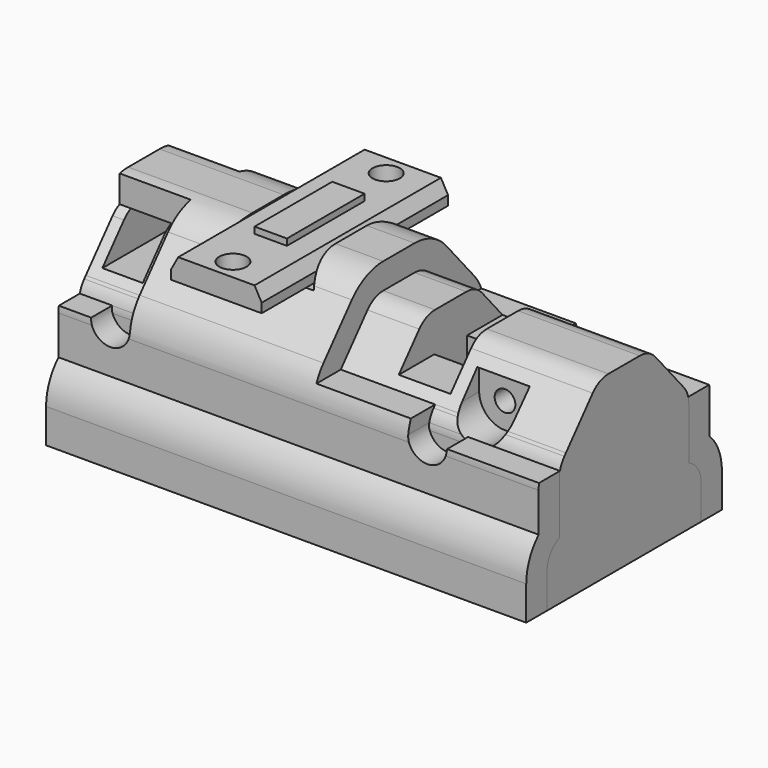
from build123d import *

# Parameters (mm, degrees)
F1_DEPTH    = 47.117
F2_T1_DEPTH = 58.7771515799
F2_T3_DEPTH = 56.5339110215
F2_T5_DEPTH = 65.2562282085
F3_T        = -2.54
F4_W        = 22.098
F4_H        = 12.7
F5_DEPTH    = 25.4
F7_DEPTH    = 25.4
F10_DEPTH   = 25.4
F12_DEPTH   = 25.4
F15_DEPTH   = 47.117
F16_W       = 3.9624000001
F16_H       = 3.9624
F17_DEPTH   = 25.4
F18_W       = 5.08
F18_H       = 6.35
F19_DEPTH   = 25.4
F20_R       = 1.016
F21_DEPTH   = 25.4
F23_R       = 1.016
F24_DEPTH   = 25.4
F26_DEPTH   = 25.4
F28_R       = 1.905
F29_DEPTH   = 25.4
F31_DEPTH   = 11.43
F32_W       = 1.5875
F32_H       = 0.635
F33_DEPTH   = 4.7625
F35_W       = 0.508
F35_H       = 2.1844
F36_DEPTH   = 12.7
F37_R       = 1.3462
F38_DEPTH   = 25.4


# Not quite as in the source:
# - a fillet or chamfer that OpenCascade refuses, or shapes differently, is made with other operations: its cross-section is extruded or revolved along the edge and cut away or added


with BuildPart() as f1:
    # F0 (on Right) → F1 (new body)
    with BuildSketch(Plane.YZ):
        Polygon((0, 6.985), (0, 0), (10.4775, 0), (12.0015, 0), (12.0015, 6.985), (10.4775, 6.985), (10.4775, 12.7), (4.2545, 19.939), (0, 19.939), align=None)
    extrude(amount=-F1_DEPTH)

    # F2: fillet of radius 5.08 on 3 edges, made by hand

    # F2_s2 → F2_t1 (cut)
    with BuildSketch(Plane.YZ.offset(-52.9470757899)):
        with BuildLine():
            ThreePointArc((5.7747186215, 18.1705824199), (4.0418518236, 19.4757758606), (1.922469684, 19.939))
            Line((1.922469684, 19.939), (4.2545, 19.939))
            Line((4.2545, 19.939), (5.7747186215, 18.1705824199))
        make_face()
    extrude(amount=F2_T1_DEPTH, mode=Mode.SUBTRACT)

    # F2_s4 → F2_t3 (cut)
    with BuildSketch(Plane.YZ.offset(-51.8254555107)):
        with BuildLine():
            ThreePointArc((9.2497489375, 14.1282002156), (10.160683001, 12.5825418311), (10.4775, 10.8166177957))
            Line((10.4775, 10.8166177957), (10.4775, 12.7))
            Line((10.4775, 12.7), (9.2497489375, 14.1282002156))
        make_face()
    extrude(amount=F2_T3_DEPTH, mode=Mode.SUBTRACT)

    # F2_s6 → F2_t5 (cut)
    with BuildSketch(Plane.YZ.offset(-56.1866141042)):
        with BuildLine():
            ThreePointArc((10.4775, 6.985), (11.6050285843, 5.3246298982), (12.0015, 3.3571543583))
            Line((12.0015, 3.3571543583), (12.0015, 6.985))
            Line((12.0015, 6.985), (10.4775, 6.985))
        make_face()
    extrude(amount=F2_T5_DEPTH, mode=Mode.SUBTRACT)

    # F3
    f3_openings = [f1.faces().sort_by_distance(p)[0] for p in [
        (0, 5.138779, 8.729827),
        (-23.5585, 0, 9.9695),
        (-47.117, 5.138779, 8.729827),
        (-23.5585, 6.00075, 0),
    ]]
    offset(amount=F3_T, openings=f3_openings, kind=Kind.INTERSECTION)

    # F4 (on Front) → F5 (cut)
    with BuildSketch(Plane.XZ):
        with Locations((-11.049, 19.05)):
            Rectangle(F4_W, F4_H)
    extrude(amount=-F5_DEPTH, mode=Mode.SUBTRACT)

    # F6 (on Front) → F7 (cut)
    with BuildSketch(Plane.XZ):
        with BuildLine():
            Line((-12.827, 17.78), (-12.827, 11.43))
            ThreePointArc((-12.827, 11.43), (-10.922, 9.525), (-9.017, 11.43))
            Line((-9.017, 11.43), (0, 11.43))
            Line((0, 11.43), (0, 17.78))
            Line((0, 17.78), (-10.922, 17.78))
            Line((-10.922, 17.78), (-12.827, 17.78))
        make_face()
    extrude(amount=-F7_DEPTH, mode=Mode.SUBTRACT)

    # F9 (on offset) → F10 (cut)
    with BuildSketch(Plane.XZ.offset(-2.9845)):
        with BuildLine():
            Line((-47.117, 11.43), (-43.942, 11.43))
            ThreePointArc((-43.942, 11.43), (-42.037, 9.525), (-40.132, 11.43))
            Line((-40.132, 11.43), (-40.132, 19.939))
            Line((-40.132, 19.939), (-42.037, 19.939))
            Line((-42.037, 19.939), (-47.117, 19.939))
            Line((-47.117, 19.939), (-47.117, 17.399))
            Line((-47.117, 17.399), (-47.117, 11.43))
        make_face()
    extrude(amount=-F10_DEPTH, mode=Mode.SUBTRACT)

    # F11 (on Front) → F12 (cut)
    with BuildSketch(Plane.XZ):
        Polygon((-26.7803559926, 19.939), (-34.9416440074, 19.939), (-36.068, 17.907), (-25.654, 17.907), align=None)
    extrude(amount=-F12_DEPTH, mode=Mode.SUBTRACT)

    # F13: F1 across plane


with BuildPart() as f1_1:
    add(f1.part)
    add(f1.part.mirror(Plane.XZ))


with BuildPart() as f15:
    # F14 (on Right) → F15 (new body, through all)
    with BuildSketch(Plane.YZ):
        with BuildLine():
            ThreePointArc((3.8485941527, 16.51479121), (2.9821607538, 17.1673879303), (1.922469684, 17.399))
            Line((1.922469684, 17.399), (0, 17.399))
            Line((0, 17.399), (0, 0))
            Line((0, 0), (9.4615, 0))
            Line((9.4615, 0), (9.4615, 3.3571543583))
            ThreePointArc((9.4615, 3.3571543583), (9.0466164674, 4.7483696544), (7.9375, 5.6851028113))
            Line((7.9375, 5.6851028113), (7.9375, 10.8166177957))
            ThreePointArc((7.9375, 10.8166177957), (7.9186362017, 11.1256036406), (7.8623249981, 11.43))
            ThreePointArc((7.8623249981, 11.43), (7.653993616, 11.9827380987), (7.3236244687, 12.4724090057))
            Line((7.3236244687, 12.4724090057), (7.1279760701, 12.7))
            Line((7.1279760701, 12.7), (3.8485941527, 16.51479121))
        make_face()
    extrude(amount=-F15_DEPTH)

    # F16 (on Front) → F17 (cut)
    with BuildSketch(Plane.XZ):
        with Locations((-44.0182000006, 15.4178)):
            Rectangle(F16_W, F16_H)
    extrude(amount=-F17_DEPTH, mode=Mode.SUBTRACT)

    # F18 (on Front) → F19 (cut)
    with BuildSketch(Plane.XZ):
        with Locations((-14.478, 16.764)):
            Rectangle(F18_W, F18_H)
    extrude(amount=-F19_DEPTH, mode=Mode.SUBTRACT)

    # F20 (on Front) → F21 (cut)
    with BuildSketch(Plane.XZ):
        with Locations((-8.128, 13.4493)):
            Circle(F20_R)
    extrude(amount=-F21_DEPTH, mode=Mode.SUBTRACT)

    # F23 (on offset) → F24 (cut)
    with BuildSketch(Plane.XZ.offset(-4.445)):
        with BuildLine():
            Line((-10.7040908762, 15.6083), (-10.6676519939, 13.4072553821))
            ThreePointArc((-10.6676519939, 13.4072553821), (-8.128, 10.9093), (-5.5883480061, 13.4072553821))
            Line((-5.5883480061, 13.4072553821), (-5.5519091238, 15.6083))
            Line((-5.5519091238, 15.6083), (-10.7040908762, 15.6083))
        make_face()
        with Locations((-8.128, 13.4493)):
            Circle(F23_R, mode=Mode.SUBTRACT)
    extrude(amount=-F24_DEPTH, mode=Mode.SUBTRACT)

    # F25 (on Top) → F26 (cut)
    with BuildSketch(Plane.XY):
        Polygon((-11.938, 0), (-11.938, 1.922469684), (-11.938, 2.0066), (-17.018, 2.0066), (-17.018, 1.922469684), (-17.018, 0), align=None)
    extrude(amount=F26_DEPTH, mode=Mode.SUBTRACT)

    # F27: F15 across plane


with BuildPart() as f15_1:
    add(f15.part)
    add(f15.part.mirror(Plane.XZ))

    # F28 (on Top) → F29 (cut)
    with BuildSketch(Plane.XY):
        with Locations((-14.478, 4.2926)):
            Circle(F28_R)
    extrude(amount=F29_DEPTH, mode=Mode.SUBTRACT)


with BuildPart() as f31:
    # F30 (on Front) → F31 (new body, symmetric)
    with BuildSketch(Plane.XZ):
        Polygon((-35.5859935677, 17.907), (-26.0344064323, 17.907), (-25.908, 17.907), (-27.118832692, 20.0914), (-34.603167308, 20.0914), (-35.814, 17.907), align=None)
    extrude(amount=F31_DEPTH, both=True)

    # F32 (on Front) → F33 (join, symmetric)
    with BuildSketch(Plane.XZ):
        with Locations((-31.65475, 20.4089)):
            Rectangle(F32_W, F32_H)
        with Locations((-30.06725, 20.4089)):
            Rectangle(F32_W, F32_H)
    extrude(amount=F33_DEPTH, both=True)

    # F35 (on Front) → F36 (cut, symmetric)
    with BuildSketch(Plane.XZ):
        with Locations((-35.56, 18.9992)):
            Rectangle(F35_W, F35_H)
        with Locations((-26.162, 18.9992)):
            Rectangle(F35_W, F35_H)
    extrude(amount=F36_DEPTH, both=True, mode=Mode.SUBTRACT)

    # F37 (on face) → F38 (cut)
    with BuildSketch(Plane(origin=(0, 0, 17.907), x_dir=(1, 0, 0), z_dir=(0, 0, -1))):
        with Locations((-30.861, -9.398)):
            Circle(F37_R)
        with Locations((-30.861, 9.398)):
            Circle(F37_R)
    extrude(amount=-F38_DEPTH, mode=Mode.SUBTRACT)


solid = Compound([f1_1.part, f15_1.part, f31.part])
